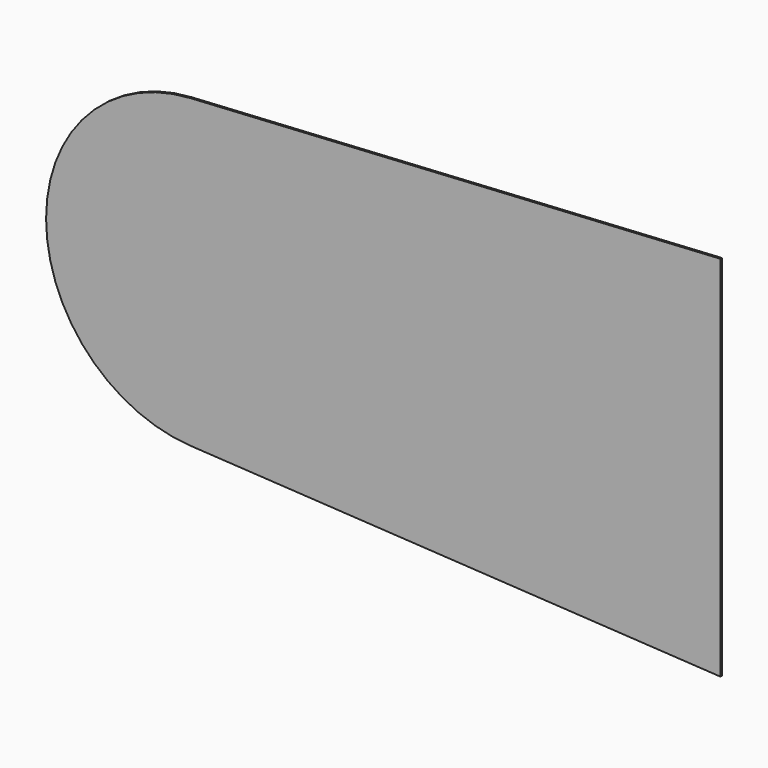
from build123d import *

# Parameters (mm, degrees)
F1_DEPTH = 0.75


# Not quite as in the source:
# - a feature names something its author has since deleted; it is built from what else it names


with BuildPart() as f1:
    # F0 (on Front) → F1 (new body, symmetric)
    with BuildSketch(Plane.XZ):
        with BuildLine():
            ThreePointArc((-432.2780955593, -124.787937418), (-339.223435441, -90.9251393865), (-300, 0))
            Line((-300, 0), (-550, 0))
            ThreePointArc((-550, 0), (-515.9251393865, -85.776564559), (-432.2780955593, -124.787937418))
        make_face()
        with BuildLine():
            Line((-550, 0), (-300, 0))
            ThreePointArc((-300, 0), (-339.223435441, 90.9251393865), (-432.2780955593, 124.787937418))
            ThreePointArc((-432.2780955593, 124.787937418), (-515.9251393865, 85.776564559), (-550, 0))
        make_face()
        with BuildLine():
            Line((0, 0), (-300, 0))
            ThreePointArc((-300, 0), (-339.223435441, -90.9251393865), (-432.2780955593, -124.787937418))
            Line((-432.2780955593, -124.787937418), (0, -150))
            Line((0, -150), (0, 0))
        make_face()
        with BuildLine():
            ThreePointArc((-432.2780955593, 124.787937418), (-339.223435441, 90.9251393865), (-300, 0))
            Line((-300, 0), (0, 0))
            Line((0, 0), (0, 150))
            Line((0, 150), (-432.2780955593, 124.787937418))
        make_face()
    extrude(amount=F1_DEPTH, both=True)


solid = f1.part
